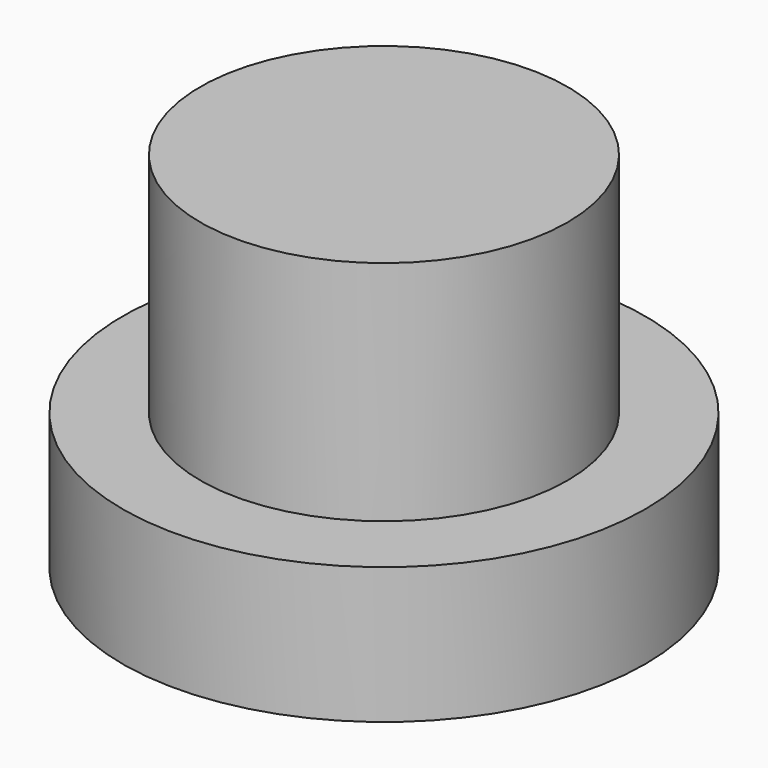
from build123d import *

# Parameters (mm, degrees)
F0_R      = 11.5
F1_DEPTH  = 6
F2_T      = -2
F3_R      = 8.0805542871
F4_DEPTH  = 10
F5_T      = 2
F7_R      = 1
F8_DEPTH  = 7
F9_R      = 0.75
F10_DEPTH = 1
F11_R     = 0.5
F12_R     = 0.0887059055
F13_DEPTH = 7


# Not quite as in the source:
# - a shell that OpenCascade refuses in one call is made with other operations: the cavity is built on its own and cut out


with BuildPart() as f1:
    # F0 (on Top) → F1 (new body)
    with BuildSketch(Plane.XY):
        with Locations((-24.4241058826, 15.6410522759)):
            Circle(F0_R)
    extrude(amount=F1_DEPTH)

    # F2
    f2_openings = [f1.faces().sort_by_distance(p)[0] for p in [
        (-24.424106, 15.641052, 0),
    ]]
    offset(amount=F2_T, openings=f2_openings)

    # F3 (on face) → F4 (join)
    with BuildSketch(Plane.XY.offset(6)):
        with Locations((-24.4241058826, 15.6410522759)):
            Circle(F3_R)
    extrude(amount=F4_DEPTH)

    # F5: shell of thickness 2, made by hand


with BuildPart() as f5_core1:
    # F5_t2: copy of F1
    add(f1.part)

    # the walls: a layer under each face that stays
    f5_faces = [f5_core1.faces().sort_by_distance(p)[0] for p in [
        (-35.9241058826, 15.6410522759, 3),
        (-32.0907725493, 7.9743856092, 0),
        (-32.0907725493, 7.9743856092, 6),
        (-33.9241058826, 15.6410522759, 2),
        (-32.5046601698, 15.6410522759, 11),
        (-24.4241058826, 15.6410522759, 16),
    ]]
    thicken(f5_faces, amount=-F5_T, mode=Mode.SUBTRACT)

    # F5_s3 → F5_t4 (revolve, cut)
    with BuildSketch(Plane.XZ.offset(-15.6410522759)):
        Polygon((-16.3235515955, 6.02), (-16.3435515955, 4), (-18.3435515955, 4), (-18.3435515955, 6), align=None)
    revolve(axis=Axis((-24.4241058826, 15.6410522759, 6), (0, 0, 1)), mode=Mode.SUBTRACT)


with BuildPart() as f1_1:
    add(f1.part)

    # what is left inside the walls is the cavity
    f5_cavity = [f5_core1.part.solids().sort_by_distance(p)[0] for p in [
        (-30.48466, 15.641052, 11.333333),
    ]]
    add(f5_cavity, mode=Mode.SUBTRACT)

    # F7 (on offset) → F8 (cut)
    with BuildSketch(Plane.XZ.offset(-29.7)):
        with Locations((-24.9341819435, 10.1343514398)):
            Circle(F7_R)
    extrude(amount=F8_DEPTH, mode=Mode.SUBTRACT)

    # F9 (on face) → F10 (join)
    with BuildSketch(Plane(origin=(0, 22.7, 0), x_dir=(-1, 0, 0), z_dir=(0, 1, 0))):
        with Locations((24.9341819435, 10.1343514398)):
            Circle(F9_R)
    extrude(amount=F10_DEPTH)

    # F11
    f11_edges = [f1_1.edges().sort_by_distance(p)[0] for p in [
        (-24.184182, 23.7, 10.134351),
    ]]
    fillet(f11_edges, radius=F11_R)

    # F12 (on face) → F13 (cut)
    with BuildSketch(Plane(origin=(0, 23.7, 0), x_dir=(-1, 0, 0), z_dir=(0, 1, 0))):
        with Locations((24.9341819435, 10.1343514398)):
            Circle(F12_R)
    extrude(amount=-F13_DEPTH, mode=Mode.SUBTRACT)


solid = f1_1.part
